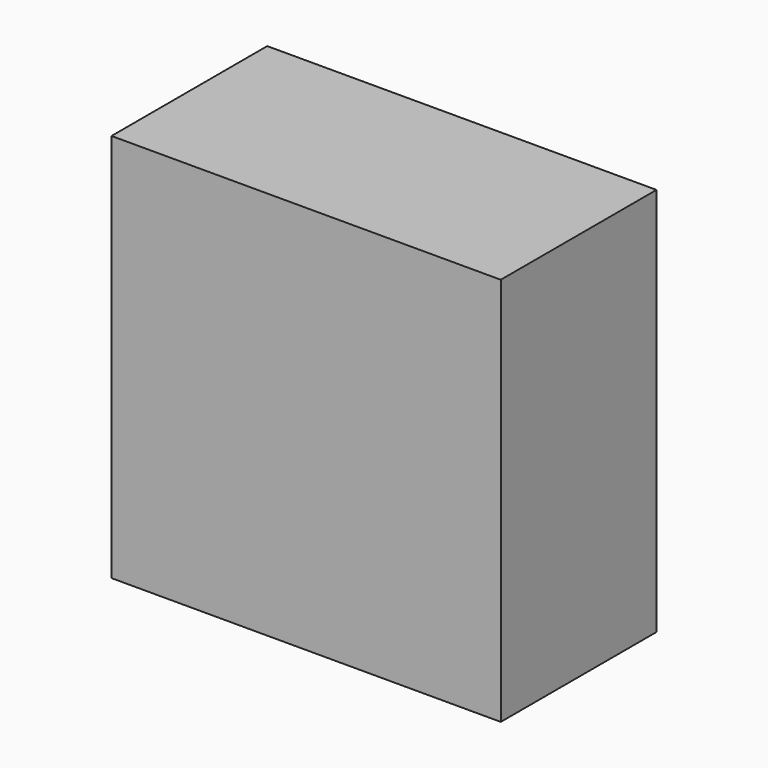
from build123d import *

# Parameters (mm, degrees)
F1_W     = 152.4
F1_H     = 152.4
F2_DEPTH = 76.2


# Not quite as in the source:
# - a variable given as a bare number and used for a length is read in inches; the dataset says mm whatever the document's units were


with BuildPart() as f2:
    # F1 (on Front) → F2 (new body)
    with BuildSketch(Plane.XZ):
        Rectangle(F1_W, F1_H)
    extrude(amount=F2_DEPTH)


solid = f2.part
